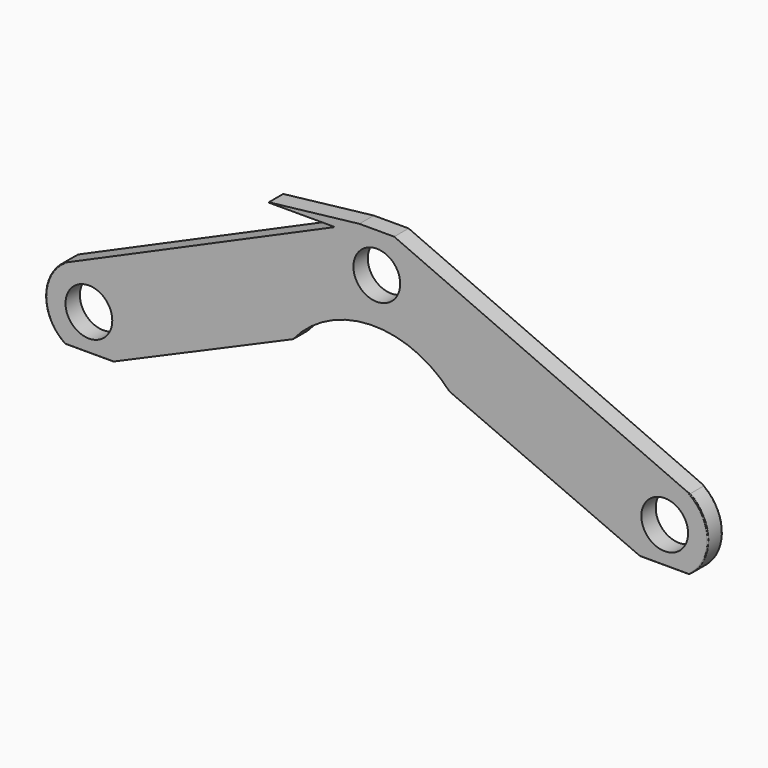
from build123d import *

# Parameters (mm, degrees)
F0_R     = 6.5
F1_DEPTH = 5
F3_R     = 0.2


# Not quite as in the source:
# - a feature of the source that left no trace in its solid (it failed there, or was rolled back) is left out


with BuildPart() as f1:
    # F0 (on Front) → F1 (new body)
    with BuildSketch(Plane.XZ):
        with BuildLine():
            Line((-11.6401047196, 31.2017867216), (-86.9632974703, -2.0251641974))
            ThreePointArc((-86.9632974703, -2.0251641974), (-91.998328651, -11.9984870467), (-86.6332495807, -21.7982132784))
            Line((-86.6332495807, -21.7982132784), (-73.3667504193, -21.7982132784))
            Line((-73.3667504193, -21.7982132784), (-23.2548427581, 0))
            ThreePointArc((-23.2548427581, 0), (-1.8189642808, 10.5340546664), (20.2171359245, 1.3213741908))
            Line((20.2171359245, 1.3213741908), (73.3667504193, -21.7982132784))
            Line((73.3667504193, -21.7982132784), (86.6332495807, -21.7982132784))
            ThreePointArc((86.6332495807, -21.7982132784), (91.998328651, -11.9984870467), (86.9632974703, -2.0251641974))
            Line((86.9632974703, -2.0251641974), (4.8428413091, 34.2017867216))
            Line((4.8428413091, 34.2017867216), (-4.8393128322, 34.2017867216))
            Line((-4.8393128322, 34.2017867216), (-30, 31.3017867216))
            Line((-30, 31.3017867216), (-30, 31.2017867216))
            Line((-30, 31.2017867216), (-11.6401047196, 31.2017867216))
        make_face()
        with Locations((-80, -11.7982132784)):
            Circle(F0_R, mode=Mode.SUBTRACT)
        with Locations((80, -11.7982132784)):
            Circle(F0_R, mode=Mode.SUBTRACT)
        with Locations((0, 23.2017867216)):
            Circle(F0_R, mode=Mode.SUBTRACT)
    extrude(amount=F1_DEPTH)

    # F3
    f3_edges = [f1.edges().sort_by_distance(p)[0] for p in [
        (80, -5, -21.798213),
        (80, 0, -21.798213),
        (-80, -5, -21.798213),
        (-80, 0, -21.798213),
        (-86.63325, -2.5, -21.798213),
        (-91.998329, 0, -11.998487),
        (-91.998329, -5, -11.998487),
        (86.63325, -2.5, -21.798213),
        (91.998329, 0, -11.998487),
        (91.998329, -5, -11.998487),
    ]]
    fillet(f3_edges, radius=F3_R)


solid = f1.part
